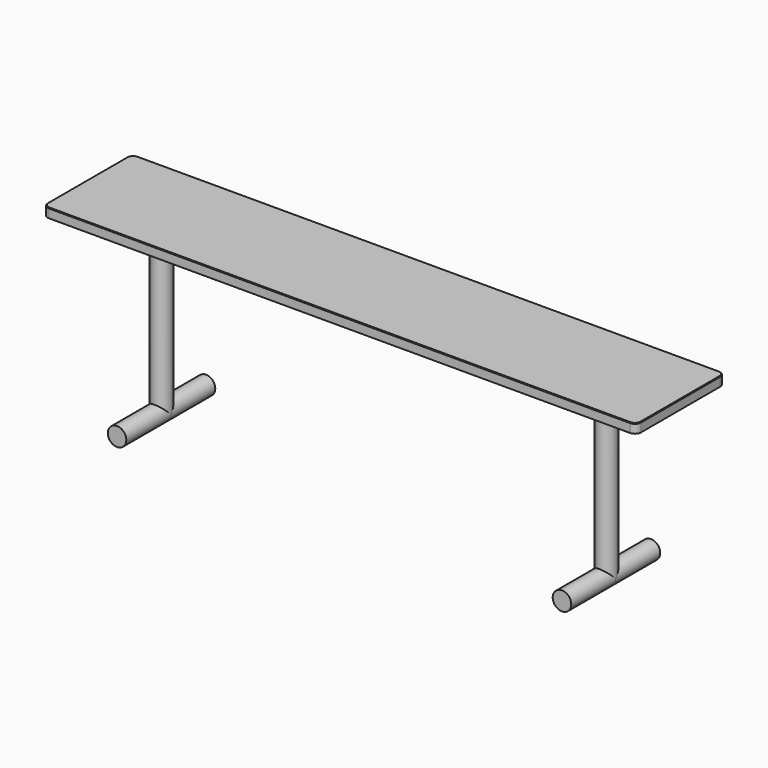
from build123d import *

# Parameters (mm, degrees)
F3_START      = 698.5
F2_W          = 2438.4
F2_H          = 457.2
F2_R          = 38.1
F3_DEPTH      = 38.1
F4_DEPTH      = 736.6
F5_R          = 38.1
F6_DEPTH      = 228.6
F6_DEPTH_BACK = 228.6
F7_R          = 25.4
F8_SIZE       = 2.54


# Not quite as in the source:
# - a variable given as a bare number and used for a length is read in inches; the dataset says mm whatever the document's units were


with BuildPart() as f3:
    # F2 (on Top) → F3 (new body)
    with BuildSketch(Plane.XY.offset(F3_START)):
        Rectangle(F2_W, F2_H)
        with Locations((-914.4, 0)):
            Circle(F2_R, mode=Mode.SUBTRACT)
        with Locations((914.4, 0)):
            Circle(F2_R, mode=Mode.SUBTRACT)
        with Locations((-914.4, 0)):
            Circle(F2_R)
        with Locations((914.4, 0)):
            Circle(F2_R)
    extrude(amount=F3_DEPTH)

    # F2 (on Top) → F4 (join)
    with BuildSketch(Plane.XY):
        with Locations((-914.4, 0)):
            Circle(F2_R)
        with Locations((914.4, 0)):
            Circle(F2_R)
    extrude(amount=F4_DEPTH)

    # F5 (on Front) → F6 (join, two sides)
    with BuildSketch(Plane.XZ) as f6_sk:
        with Locations((-914.4, 0)):
            Circle(F5_R)
        with Locations((914.4, 0)):
            Circle(F5_R)
    extrude(amount=F6_DEPTH)
    extrude(f6_sk.sketch, amount=-F6_DEPTH_BACK)

    # F7
    f7_edges = [f3.edges().sort_by_distance(p)[0] for p in [
        (1219.2, -228.6, 717.55),
        (1219.2, 228.6, 717.55),
        (-1219.2, -228.6, 717.55),
        (-1219.2, 228.6, 717.55),
    ]]
    fillet(f7_edges, radius=F7_R)

    # F8
    f8_edges = [f3.edges().sort_by_distance(p)[0] for p in [
        (-1219.2, 0, 736.6),
        (-1211.760512, 221.160512, 736.6),
        (0, 228.6, 736.6),
        (-1211.760512, -221.160512, 736.6),
        (0, -228.6, 736.6),
        (1219.2, 0, 736.6),
        (1211.760512, 221.160512, 736.6),
        (1211.760512, -221.160512, 736.6),
    ]]
    chamfer(f8_edges, length=F8_SIZE)


solid = f3.part
